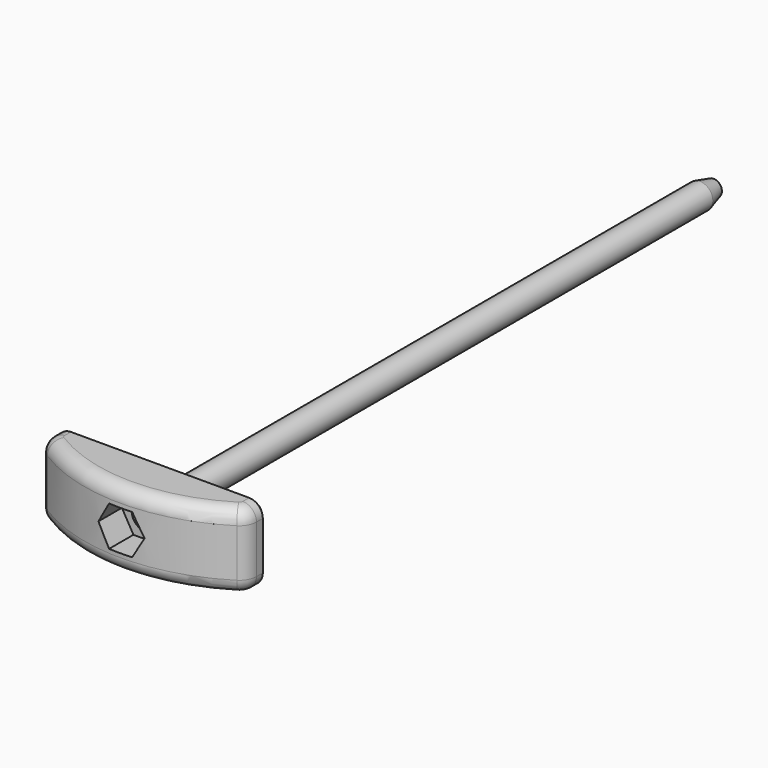
from build123d import *

# Parameters (mm, degrees)
F0_R      = 4.7625
F1_DEPTH  = 254
F2_SIZE2  = 1.7014773719
F2_SIZE   = 6.35
F4_DEPTH  = 13.97
F7_DEPTH  = 15.875
F8_R      = 6.35
F9_R      = 4.8895
F10_DEPTH = 263.526
F11_R     = 5.08
F12_SIZE  = 2.54


# Not quite as in the source:
# - a feature names something its author has since deleted; it is built from what else it names


with BuildPart() as f1:
    # F0 (on Front) → F1 (new body)
    with BuildSketch(Plane.XZ):
        Circle(F0_R)
    extrude(amount=-F1_DEPTH)

    # F2
    f2_edges = [f1.edges().sort_by_distance(p)[0] for p in [
        (-4.7625, 254, 0),
    ]]
    f2_side = f1.faces().sort_by_distance((-4.7625, 127, 0))[0]
    chamfer(f2_edges, length=F2_SIZE, length2=F2_SIZE2, reference=f2_side)


with BuildPart() as f4:
    # F3 (on Top) → F4 (new body, symmetric)
    with BuildSketch(Plane.XY):
        with BuildLine():
            Line((-38.1, 0), (-38.1, -8.89))
            ThreePointArc((-38.1, -8.89), (0, -20.9310323016), (38.1, -8.89))
            Line((38.1, -8.89), (38.1, 0))
            Line((38.1, 0), (-38.1, 0))
        make_face()
    extrude(amount=F4_DEPTH, both=True)

    # F6 (on offset) → F7 (cut)
    with BuildSketch(Plane.XZ.offset(25.4)):
        Polygon((8.5495182562, 0), (4.2747591281, 7.4041), (-4.2747591281, 7.4041), (-8.5495182562, 0), (-4.2747591281, -7.4041), (4.2747591281, -7.4041), align=None)
    extrude(amount=-F7_DEPTH, mode=Mode.SUBTRACT)

    # F8
    f8_edges = [f4.edges().sort_by_distance(p)[0] for p in [
        (38.1, -8.89, 0),
        (-38.1, -8.89, 0),
    ]]
    fillet(f8_edges, radius=F8_R)

    # F9 (on face) → F10 (cut, through all)
    with BuildSketch(Plane.XZ.offset(9.525)):
        Circle(F9_R)
    extrude(amount=-F10_DEPTH, mode=Mode.SUBTRACT)

    # F11
    f11_edges = [f4.edges().sort_by_distance(p)[0] for p in [
        (0, -20.931032, -13.97),
        (0, -20.931032, 13.97),
        (-37.3033, -8.562348, -13.97),
        (37.3033, -8.562348, -13.97),
        (-37.3033, -8.562348, 13.97),
        (37.3033, -8.562348, 13.97),
    ]]
    fillet(f11_edges, radius=F11_R)

    # F12
    f12_edges = [f4.edges().sort_by_distance(p)[0] for p in [
        (0, 0, -13.97),
        (-38.1, 0, 0),
        (0, 0, 13.97),
        (38.1, 0, 0),
        (-36.612102, 0, 12.482102),
        (-36.612102, 0, -12.482102),
        (36.612102, 0, -12.482102),
        (36.612102, 0, 12.482102),
    ]]
    chamfer(f12_edges, length=F12_SIZE)


solid = Compound([f1.part, f4.part])
